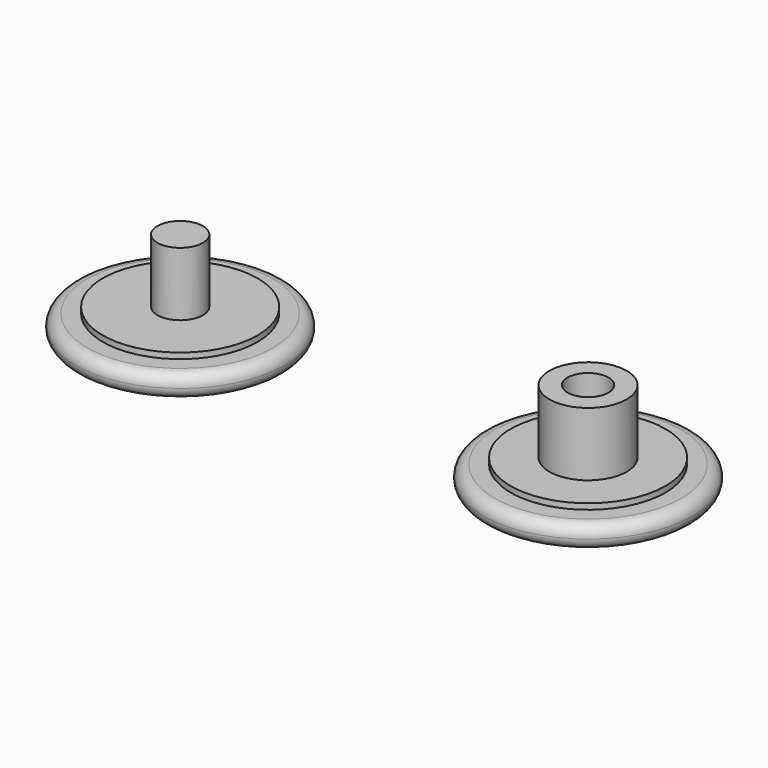
from build123d import *

# Parameters (mm, degrees)
F0_R      = 11.5
F0_R_2    = 8.5
F1_DEPTH  = 2.54
F0_R_3    = 4.25
F2_DEPTH  = 3.175
F3_DEPTH  = 10.175
F4_R      = 1.26999
F5_R      = 11.5
F5_R_2    = 8.5
F6_DEPTH  = 2.54
F5_R_3    = 2.5
F7_DEPTH  = 3.175
F8_DEPTH  = 10.175
F9_R      = 2.25
F10_DEPTH = 7
F11_R     = 1.26999


# Not quite as in the source:
# - a fillet or chamfer is up to 0.001 mm smaller than in the source, because OpenCascade refuses the exact size


with BuildPart() as f1:
    # F0 (on Top) → F1 (new body)
    with BuildSketch(Plane.XY):
        Circle(F0_R)
        Circle(F0_R_2, mode=Mode.SUBTRACT)
    extrude(amount=F1_DEPTH)

    # F0 (on Top) → F2 (join)
    with BuildSketch(Plane.XY):
        Circle(F0_R_2)
        Circle(F0_R_3, mode=Mode.SUBTRACT)
    extrude(amount=F2_DEPTH)

    # F0 (on Top) → F3 (join)
    with BuildSketch(Plane.XY):
        Circle(F0_R_3)
    extrude(amount=F3_DEPTH)

    # F4 (radius 1.27 in the source; OpenCascade refuses exactly that, so slightly less here)
    f4_edges = [f1.edges().sort_by_distance(p)[0] for p in [
        (-11.5, 0, 2.54),
        (-11.5, 0, 0),
    ]]
    fillet(f4_edges, radius=F4_R)

    # F9 (on face) → F10 (cut)
    with BuildSketch(Plane.XY.offset(10.175)):
        Circle(F9_R)
    extrude(amount=-F10_DEPTH, mode=Mode.SUBTRACT)


with BuildPart() as f6:
    # F5 (on Top) → F6 (new body)
    with BuildSketch(Plane.XY):
        with Locations((-44.7985892718, 0)):
            Circle(F5_R)
        with Locations((-44.7985892718, 0)):
            Circle(F5_R_2, mode=Mode.SUBTRACT)
    extrude(amount=F6_DEPTH)

    # F5 (on Top) → F7 (join)
    with BuildSketch(Plane.XY):
        with Locations((-44.7985892718, 0)):
            Circle(F5_R_2)
        with Locations((-44.7985892718, 0)):
            Circle(F5_R_3, mode=Mode.SUBTRACT)
    extrude(amount=F7_DEPTH)

    # F5 (on Top) → F8 (join)
    with BuildSketch(Plane.XY):
        with Locations((-44.7985892718, 0)):
            Circle(F5_R_3)
    extrude(amount=F8_DEPTH)

    # F11 (radius 1.27 in the source; OpenCascade refuses exactly that, so slightly less here)
    f11_edges = [f6.edges().sort_by_distance(p)[0] for p in [
        (-56.298589, 0, 2.54),
        (-56.298589, 0, 0),
    ]]
    fillet(f11_edges, radius=F11_R)


solid = Compound([f1.part, f6.part])
